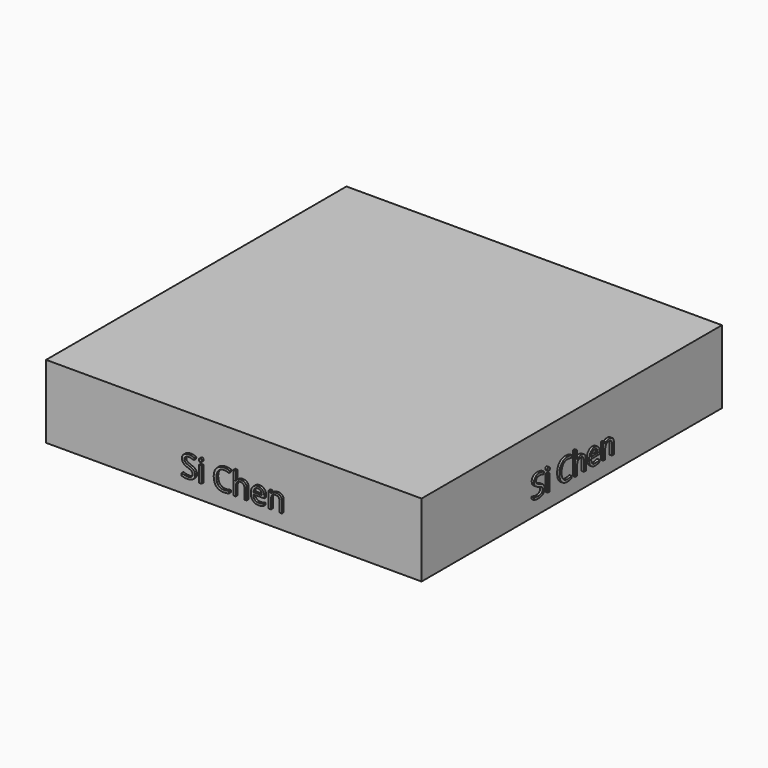
from build123d import *

# Parameters (mm, degrees)
F0_W         = 164.4
F0_H         = 164.4
F0_W_2       = 154.4
F0_H_2       = 154.4
F1_DEPTH     = 7
F0_W_3       = 152.4
F0_H_3       = 152.4
F2_DEPTH     = 25
F3_TEXT_SIZE = 13.1000901713
F4_DEPTH     = 1
F5_TEXT_SIZE = 13.1000901713
F6_DEPTH     = 1
F7_TEXT_SIZE = 13.1000901713
F8_DEPTH     = 1
F9_TEXT_SIZE = 13.1000901713
F10_DEPTH    = 1


# Not quite as in the source:
# - Text() gives the source's letters only with a copy of the font that has no kerning and outlines rounded to 1/6400 em; it was checked with that copy


with BuildPart() as f1:
    # F0 (on Top) → F1 (new body)
    with BuildSketch(Plane.XY):
        with Locations((24.1863926325, -35.0005550941)):
            Rectangle(F0_W, F0_H)
        with Locations((24.1863926325, -35.0005550941)):
            Rectangle(F0_W_2, F0_H_2, mode=Mode.SUBTRACT)
    extrude(amount=-F1_DEPTH)

    # F0 (on Top) → F2 (join)
    with BuildSketch(Plane.XY):
        with Locations((24.1863926325, -35.0005550941)):
            Rectangle(F0_W, F0_H)
        with Locations((24.1863926325, -35.0005550941)):
            Rectangle(F0_W_2, F0_H_2, mode=Mode.SUBTRACT)
        with Locations((24.1863926325, -35.0005550941)):
            Rectangle(F0_W_2, F0_H_2)
        with Locations((24.1863926325, -35.0005550941)):
            Rectangle(F0_W_3, F0_H_3, mode=Mode.SUBTRACT)
        with Locations((24.1863926325, -35.0005550941)):
            Rectangle(F0_W_3, F0_H_3)
    extrude(amount=F2_DEPTH)

    # F3 (on face) → F4 (join)
    with BuildSketch(Plane.XZ.offset(117.2005550941)):
        with Locations((1.4863926325, 0)):
            Text('Si Chen', F3_TEXT_SIZE, font='Open Sans', text_align=(TextAlign.LEFT, TextAlign.BOTTOM))
    extrude(amount=F4_DEPTH)

    # F5 (on face) → F6 (join)
    with BuildSketch(Plane(origin=(-58.0136073675, 0, 0), x_dir=(0, -1, 0), z_dir=(-1, 0, 0))):
        with Locations((12.3005550941, 6)):
            Text('Si Chen', F5_TEXT_SIZE, font='Open Sans', text_align=(TextAlign.LEFT, TextAlign.BOTTOM))
    extrude(amount=F6_DEPTH)

    # F7 (on face) → F8 (join)
    with BuildSketch(Plane.YZ.offset(106.3863926325)):
        with Locations((-57.7005550941, 0)):
            Text('Si Chen', F7_TEXT_SIZE, font='Open Sans', text_align=(TextAlign.LEFT, TextAlign.BOTTOM))
    extrude(amount=F8_DEPTH)

    # F9 (on face) → F10 (join)
    with BuildSketch(Plane(origin=(0, 47.1994449059, 0), x_dir=(-1, 0, 0), z_dir=(0, 1, 0))):
        with Locations((-46.8863926325, 6)):
            Text('Si Chen', F9_TEXT_SIZE, font='Open Sans', text_align=(TextAlign.LEFT, TextAlign.BOTTOM))
    extrude(amount=F10_DEPTH)


solid = f1.part
